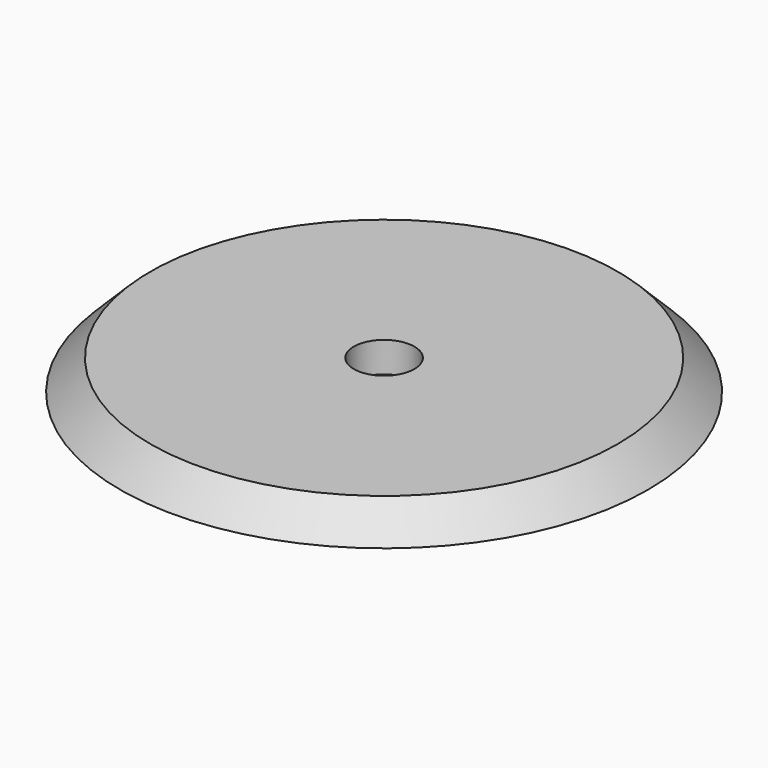
from build123d import *

# Parameters (mm, degrees)
F0_R     = 43.5
F0_R_2   = 5
F1_DEPTH = 5
F2_SIZE  = 4.99999


# Not quite as in the source:
# - a fillet or chamfer is up to 0.001 mm smaller than in the source, because OpenCascade refuses the exact size


with BuildPart() as f1:
    # F0 (on Top) → F1 (new body)
    with BuildSketch(Plane.XY):
        Circle(F0_R)
        Circle(F0_R_2, mode=Mode.SUBTRACT)
    extrude(amount=F1_DEPTH)

    # F2 (size 5 in the source; OpenCascade refuses exactly that, so slightly less here)
    f2_edges = [f1.edges().sort_by_distance(p)[0] for p in [
        (-43.5, 0, 5),
    ]]
    chamfer(f2_edges, length=F2_SIZE)


solid = f1.part
